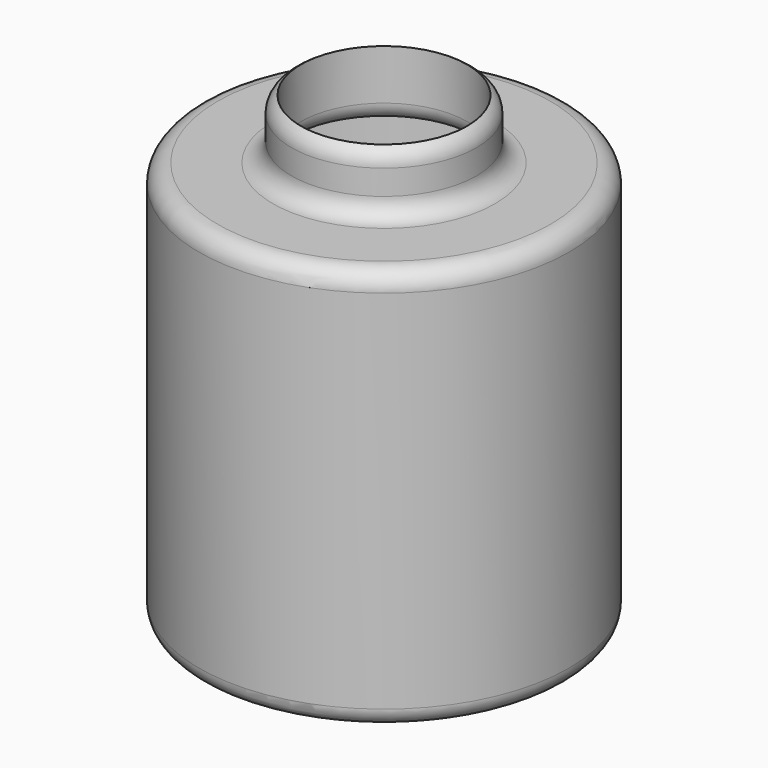
from build123d import *


# Not quite as in the source:
# - a fillet or chamfer that OpenCascade refuses, or shapes differently, is made with other operations: its cross-section is extruded or revolved along the edge and cut away or added


with BuildPart() as f1:
    # F0 (on Front) → F1 (revolve)
    with BuildSketch(Plane.XZ):
        Polygon((25.4, 63.5), (22.844016552, 63.5), (22.844016552, 44.6444414556), (48.6258789897, 44.6444414556), (48.6258789897, -61.2174496055), (1.9450800028, -61.2174496055), (0, -61.2174496055), (0, -63.5), (50.8, -63.5), (50.8, 47.1835695207), (25.4, 47.1835695207), (25.4, 62.8089383245), align=None)
    revolve(axis=Axis((0, 0, -31.75), (0, 0, -1)))

    # F2: fillet of radius 5.08 on 7 edges, made by hand

    # F2_s1 → F2_t2 (revolve)
    with BuildSketch(Plane.XZ):
        with BuildLine():
            ThreePointArc((30.48, 47.1835695207), (26.8878975516, 48.6714670723), (25.4, 52.2635695207))
            Line((25.4, 52.2635695207), (25.4, 47.1835695207))
            Line((25.4, 47.1835695207), (30.48, 47.1835695207))
        make_face()
    revolve(axis=Axis((0, 0, 47.1835695207), (0, 0, -1)))

    # F2_s3 → F2_t4 (revolve)
    with BuildSketch(Plane.XZ):
        with BuildLine():
            ThreePointArc((48.6258789897, -56.1374496055), (47.1379814381, -59.7295520539), (43.5458789897, -61.2174496055))
            Line((43.5458789897, -61.2174496055), (48.6258789897, -61.2174496055))
            Line((48.6258789897, -61.2174496055), (48.6258789897, -56.1374496055))
        make_face()
    revolve(axis=Axis((0, 0, -61.2174496055), (0, 0, -1)))

    # F2_s5 → F2_t6 (revolve, cut)
    with BuildSketch(Plane.XZ):
        with BuildLine():
            ThreePointArc((45.72, 47.1835695207), (49.3121024484, 45.6956719691), (50.8, 42.1035695207))
            Line((50.8, 42.1035695207), (50.8, 47.1835695207))
            Line((50.8, 47.1835695207), (45.72, 47.1835695207))
        make_face()
    revolve(axis=Axis((0, 0, 47.1835695207), (0, 0, -1)), mode=Mode.SUBTRACT)

    # F2_s7 → F2_t8 (revolve, cut)
    with BuildSketch(Plane.XZ):
        with BuildLine():
            ThreePointArc((25.4, 59.0914015328), (24.7147926051, 61.6393807238), (22.844016552, 63.5))
            Line((22.844016552, 63.5), (25.4, 63.5))
            Line((25.4, 63.5), (25.4, 59.0914015328))
        make_face()
    revolve(axis=Axis((0, 0, 63.5), (0, 0, -1)), mode=Mode.SUBTRACT)

    # F2_s9 → F2_t10 (revolve, cut)
    with BuildSketch(Plane.XZ):
        with BuildLine():
            ThreePointArc((22.844016552, 49.7244414556), (24.3319141035, 46.1323390072), (27.924016552, 44.6444414556))
            Line((27.924016552, 44.6444414556), (22.844016552, 44.6444414556))
            Line((22.844016552, 44.6444414556), (22.844016552, 49.7244414556))
        make_face()
    revolve(axis=Axis((0, 0, 44.6444414556), (0, 0, -1)), mode=Mode.SUBTRACT)

    # F2_s11 → F2_t12 (revolve, cut)
    with BuildSketch(Plane.XZ):
        with BuildLine():
            ThreePointArc((50.8, -58.42), (49.3121024484, -62.0121024484), (45.72, -63.5))
            Line((45.72, -63.5), (50.8, -63.5))
            Line((50.8, -63.5), (50.8, -58.42))
        make_face()
    revolve(axis=Axis((0, 0, -63.5), (0, 0, -1)), mode=Mode.SUBTRACT)


solid = f1.part
